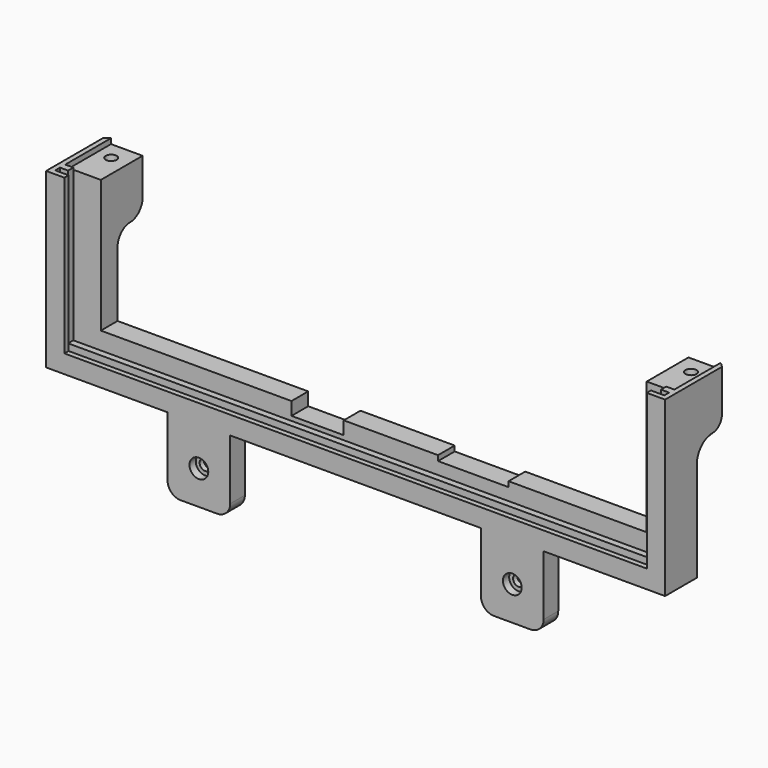
from build123d import *

# Parameters (mm, degrees)
F1_DEPTH  = 8
F3_DEPTH  = 1.9
F5_DEPTH  = 2.5
F7_DEPTH  = 2.3
F9_W      = 14
F9_H      = 22
F10_DEPTH = 12
F11_DEPTH = 2
F12_W     = 12.1
F12_H     = 20
F13_W     = 12.1
F13_H     = 20
F14_DEPTH = 2
F17_R     = 5.99999
F18_R     = 5.99999
F19_DEPTH = 10
F20_DEPTH = 25
F22_R     = 2.1
F21_R     = 2.1
F23_DEPTH = 10
F24_SIZE  = 1.5
F25_W     = 24
F25_H     = 8
F26_DEPTH = 28
F28_R     = 4.1
F27_R     = 4.1
F29_DEPTH = 3
F30_R     = 2.1
F31_DEPTH = 28.701
F32_R     = 3.6
F33_DEPTH = 3
F34_R     = 5
F35_W     = 20
F35_H     = 8
F36_DEPTH = 5
F37_SIZE  = 1
F38_W     = 27
F38_H     = 8
F39_DEPTH = 2


# Not quite as in the source:
# - a fillet or chamfer is up to 0.001 mm smaller than in the source, because OpenCascade refuses the exact size
# - a feature names something its author has since deleted; it is built from what else it names


with BuildPart() as f1:
    # F0 (on Front) → F1 (new body)
    with BuildSketch(Plane.XZ):
        Polygon((-118.5, 0), (118.5, 0), (118.5, 66.23), (104.5, 66.23), (104.5, 13.43), (-104.5, 13.43), (-104.5, 66.23), (-118.5, 66.23), align=None)
    extrude(amount=F1_DEPTH)

    # F2 (on face) → F3 (join)
    with BuildSketch(Plane.XZ.offset(8)):
        Polygon((-116.6, 66.23), (-118.5, 66.23), (-118.5, 0), (118.5, 0), (118.5, 66.23), (116.6, 66.23), (116.6, 3.43), (-116.6, 3.43), align=None)
    extrude(amount=F3_DEPTH)

    # F4 (on face) → F5 (join)
    with BuildSketch(Plane.XZ.offset(9.9)):
        Polygon((-113.5, 66.23), (-118.5, 66.23), (-118.5, 0), (118.5, 0), (118.5, 66.23), (113.5, 66.23), (113.5, 8), (-113.5, 8), align=None)
    extrude(amount=F5_DEPTH)

    # F6 (on face) → F7 (join)
    with BuildSketch(Plane.XZ.offset(12.4)):
        Polygon((-116.6, 66.23), (-118.5, 66.23), (-118.5, 0), (118.5, 0), (118.5, 66.23), (116.6, 66.23), (116.6, 3.43), (-116.6, 3.43), align=None)
    extrude(amount=F7_DEPTH)

    # F9 (on face) → F10 (join)
    with BuildSketch(Plane(origin=(0, 0, 0), x_dir=(-1, 0, 0), z_dir=(0, 1, 0))):
        with Locations((111.5, 55.23)):
            Rectangle(F9_W, F9_H)
        with Locations((-111.5, 55.23)):
            Rectangle(F9_W, F9_H)
    extrude(amount=F10_DEPTH)

    # F8 (on face) → F11 (join)
    with BuildSketch(Plane.XZ.offset(14.7)):
        Polygon((-111.5, 66.23), (-118.5, 66.23), (-118.5, 0), (118.5, 0), (118.5, 66.23), (111.5, 66.23), (111.5, 7), (-111.5, 7), align=None)
    extrude(amount=F11_DEPTH)

    # F12 (on face) + F13 (on face) → F14 (cut)
    with BuildSketch(Plane.XY.offset(66.23)):
        with Locations((-110.55, 2)):
            Rectangle(F12_W, F12_H)
    with BuildSketch(Plane.XY.offset(66.23)):
        with Locations((110.55, 2)):
            Rectangle(F13_W, F13_H)
    extrude(amount=-F14_DEPTH, mode=Mode.SUBTRACT)

    # F17 (radius 6 in the source; OpenCascade refuses exactly that, so slightly less here)
    f17_edges = [f1.edges().sort_by_distance(p)[0] for p in [
        (-111.5, 0, 44.23),
        (-111.5, 12, 44.23),
    ]]
    fillet(f17_edges, radius=F17_R)

    # F18 (radius 6 in the source; OpenCascade refuses exactly that, so slightly less here)
    f18_edges = [f1.edges().sort_by_distance(p)[0] for p in [
        (111.5, 0, 44.23),
        (111.5, 12, 44.23),
    ]]
    fillet(f18_edges, radius=F18_R)

    # F15 (on face) + F16 (on face) → F19 (cut)
    with BuildSketch(Plane(origin=(0, 0, 44.23), x_dir=(1, 0, 0), z_dir=(0, 0, -1))):
        Polygon((111, -1.1430780618), (107.4, -3.2215390309), (107.4, -7.3784609691), (111, -9.4569219382), (114.6, -7.3784609691), (114.6, -3.2215390309), align=None)
    with BuildSketch(Plane(origin=(0, 0, 44.23), x_dir=(1, 0, 0), z_dir=(0, 0, -1))):
        Polygon((-107.4, -7.3784609691), (-107.4, -3.2215390309), (-111, -1.1430780618), (-114.6, -3.2215390309), (-114.6, -7.3784609691), (-111, -9.4569219382), align=None)
    extrude(amount=-F19_DEPTH, mode=Mode.SUBTRACT)

    # F15 (on face) + F16 (on face) → F20 (cut)
    with BuildSketch(Plane(origin=(0, 0, 44.23), x_dir=(1, 0, 0), z_dir=(0, 0, -1))):
        Polygon((111, -1.1430780618), (107.4, -3.2215390309), (107.4, -7.3784609691), (111, -9.4569219382), (114.6, -7.3784609691), (114.6, -3.2215390309), align=None)
    with BuildSketch(Plane(origin=(0, 0, 44.23), x_dir=(1, 0, 0), z_dir=(0, 0, -1))):
        Polygon((-107.4, -7.3784609691), (-107.4, -3.2215390309), (-111, -1.1430780618), (-114.6, -3.2215390309), (-114.6, -7.3784609691), (-111, -9.4569219382), align=None)
    extrude(amount=F20_DEPTH, mode=Mode.SUBTRACT)

    # F22 (on face) + F21 (on face) → F23 (cut, through all)
    with BuildSketch(Plane.XY.offset(64.23)):
        with Locations((111, 5.1)):
            Circle(F22_R)
    with BuildSketch(Plane.XY.offset(64.23)):
        with Locations((-111, 5.1)):
            Circle(F21_R)
    extrude(amount=-F23_DEPTH, mode=Mode.SUBTRACT)

    # F24
    f24_edges = [f1.edges().sort_by_distance(p)[0] for p in [
        (118.5, 0, 19.115005),
        (-118.5, 0, 19.115005),
        (0, 0, 0),
        (118.5, 12, 58.229995),
        (118.5, 10.242644, 45.987356),
        (118.5, 6, 44.23),
        (118.5, 1.757356, 42.472644),
        (-118.5, 1.757356, 42.472644),
        (-118.5, 6, 44.23),
        (-118.5, 10.242644, 45.987356),
        (-118.5, 12, 58.229995),
    ]]
    chamfer(f24_edges, length=F24_SIZE)

    # F25 (on face) → F26 (join)
    with BuildSketch(Plane(origin=(0, 0, 0), x_dir=(1, 0, 0), z_dir=(0, 0, -1))):
        with Locations((-60, 12.7)):
            Rectangle(F25_W, F25_H)
        with Locations((60, 12.7)):
            Rectangle(F25_W, F25_H)
    extrude(amount=F26_DEPTH)

    # F28 (on face) + F27 (on face) → F29 (cut)
    with BuildSketch(Plane(origin=(0, -8.7, 0), x_dir=(-1, 0, 0), z_dir=(0, 1, 0))):
        with Locations((-60, -15)):
            Circle(F28_R)
    with BuildSketch(Plane(origin=(0, -8.7, 0), x_dir=(-1, 0, 0), z_dir=(0, 1, 0))):
        with Locations((60, -15)):
            Circle(F27_R)
    extrude(amount=-F29_DEPTH, mode=Mode.SUBTRACT)

    # F30 (on face) → F31 (cut, through all)
    with BuildSketch(Plane.XZ.offset(16.7)):
        with Locations((-60, -15)):
            Circle(F30_R)
        with Locations((60, -15)):
            Circle(F30_R)
    extrude(amount=-F31_DEPTH, mode=Mode.SUBTRACT)

    # F32 (on face) → F33 (cut)
    with BuildSketch(Plane.XZ.offset(16.7)):
        with Locations((-60, -15)):
            Circle(F32_R)
        with Locations((60, -15)):
            Circle(F32_R)
    extrude(amount=-F33_DEPTH, mode=Mode.SUBTRACT)

    # F34
    f34_edges = [f1.edges().sort_by_distance(p)[0] for p in [
        (-72, -12.7, -28),
        (-48, -12.7, -28),
        (48, -12.7, -28),
        (72, -12.7, -28),
    ]]
    fillet(f34_edges, radius=F34_R)

    # F35 (on face) → F36 (cut)
    with BuildSketch(Plane.XY.offset(13.43)):
        with Locations((-21.5, -4)):
            Rectangle(F35_W, F35_H)
    extrude(amount=-F36_DEPTH, mode=Mode.SUBTRACT)

    # F37
    f37_edges = [f1.edges().sort_by_distance(p)[0] for p in [
        (-72, -8.7, -11.5),
        (72, -8.7, -11.5),
        (48, -8.7, -11.5),
        (-48, -8.7, -11.5),
        (-70.535534, -8.7, -26.535534),
        (-60, -8.7, -28),
        (-49.464466, -8.7, -26.535534),
        (49.464466, -8.7, -26.535534),
        (60, -8.7, -28),
        (70.535534, -8.7, -26.535534),
    ]]
    chamfer(f37_edges, length=F37_SIZE)

    # F38 (on face) → F39 (cut)
    with BuildSketch(Plane.XY.offset(13.43)):
        with Locations((38.1, -4)):
            Rectangle(F38_W, F38_H)
    extrude(amount=-F39_DEPTH, mode=Mode.SUBTRACT)


solid = f1.part
